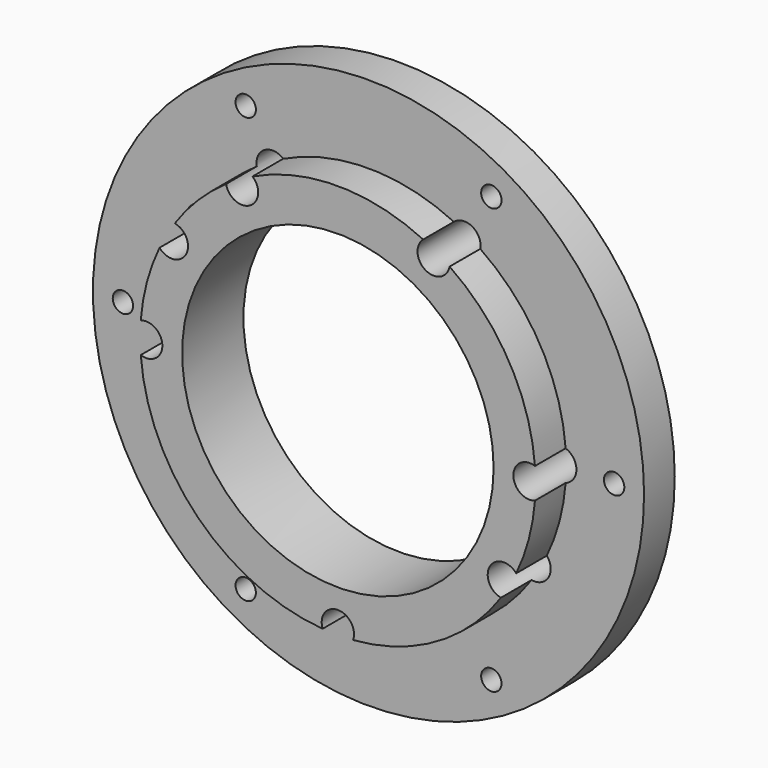
from build123d import *

# Parameters (mm, degrees)
F0_R            = 115
F1_DEPTH        = 16
F2_R            = 82.5
F3_DEPTH        = 16
F4_R            = 65
F5_DEPTH        = 32.001
F7_D            = 13.5
F9_D            = 8.5
F9_COPIES_COUNT = 6


# Not quite as in the source:
# - a pattern or mirror of a feature is missing from the dataset's text; its kind, count and spacing are read off the source's solid


with BuildPart() as f1:
    # F0 (on Front) → F1 (new body)
    with BuildSketch(Plane.XZ):
        Circle(F0_R)
    extrude(amount=F1_DEPTH)

    # F2 (on face) → F3 (join)
    with BuildSketch(Plane.XZ.offset(16)):
        Circle(F2_R)
    extrude(amount=F3_DEPTH)

    # F4 (on face) → F5 (cut, through all)
    with BuildSketch(Plane.XZ.offset(32)):
        Circle(F4_R)
    extrude(amount=-F5_DEPTH, mode=Mode.SUBTRACT)

    # F7 (through all)
    with Locations(Plane.XZ.offset(32)):
        with Locations((40, 69.2820323028), (80, 0), (69.2820323028, -40), (0, -80), (-80, 0), (-69.2820323028, 40), (-40, 69.2820323028)):
            Hole(F7_D / 2)

    # F9 (through all)
    with Locations(Plane.XZ.offset(16)):
        with Locations((51.25, 88.7676038879)):
            f9 = Hole(F9_D / 2)

    # F9_copies: F9 ×6 about axis
    f9_copies_axis = Axis((0, 0, 0), (0, 1, 0))
    for i in range(1, F9_COPIES_COUNT):
        add(f9.rotate(f9_copies_axis, i * 360 / F9_COPIES_COUNT), mode=Mode.SUBTRACT)


solid = f1.part
